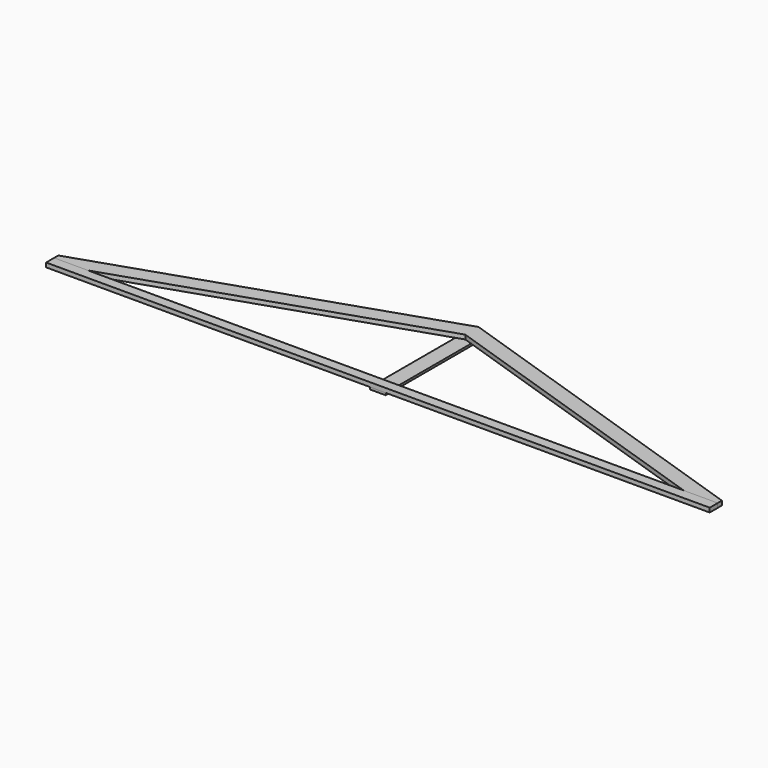
from build123d import *

# Parameters (mm, degrees)
F0_W     = 5892.8
F0_H     = 88.9
F1_DEPTH = 38.1
F2_W     = 139.7
F2_H     = 1092.2
F3_DEPTH = 19.05
F5_DEPTH = 38.1
F6_W     = 5892.8
F6_H     = 88.9
F7_DEPTH = 38.101


with BuildPart() as f1:
    # F0 (on Top) → F1 (new body)
    with BuildSketch(Plane.XY):
        with Locations((0, 44.45)):
            Rectangle(F0_W, F0_H)
    extrude(amount=F1_DEPTH)


with BuildPart() as f3:
    # F2 (on Top) → F3 (new body)
    with BuildSketch(Plane.XY):
        with Locations((0, 546.1)):
            Rectangle(F2_W, F2_H)
    extrude(amount=-F3_DEPTH)


with BuildPart() as f5:
    # F4 (on face) → F5 (new body)
    with BuildSketch(Plane.XY.offset(38.1)):
        Polygon((-2946.4, 135.4637424996), (-2946.4, 0), (-2911.0210121782, 0), (0, 970.3432264478), (0, 1117.6), align=None)
        Polygon((2946.4, 135.4637424996), (0, 1117.6), (0, 970.3432264478), (2911.0210121782, 0), (2946.4, 0), align=None)
    extrude(amount=-F5_DEPTH)

    # F6 (on face) → F7 (cut, through all)
    with BuildSketch(Plane(origin=(0, 0, 0), x_dir=(1, 0, 0), z_dir=(0, 0, -1))):
        with Locations((0, -44.45)):
            Rectangle(F6_W, F6_H)
    extrude(amount=-F7_DEPTH, mode=Mode.SUBTRACT)


solid = Compound([f1.part, f3.part, f5.part])
